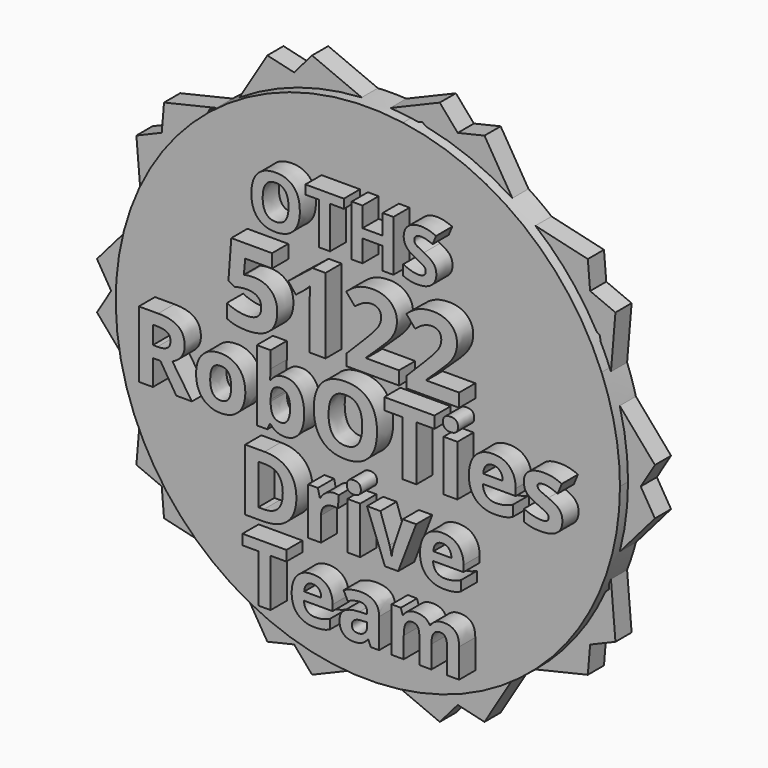
from build123d import *

# Parameters (mm, degrees)
F1_DEPTH       = 7.62
F3_DEPTH       = 5.08
F4_TEXT_SIZE   = 17.9359663485
F4_TEXT_SIZE_2 = 26.5140358048
F4_TEXT_SIZE_3 = 23.3947377031
F5_DEPTH       = 5.08
F6_DEPTH       = 12.7
F7_TEXT_SIZE   = 21.7276495985
F7_TEXT_SIZE_2 = 20.4692439487
F8_DEPTH       = 12.7


# Not quite as in the source:
# - Text() gives the source's letters only with a copy of the font that has no kerning and outlines rounded to 1/6400 em; it was checked with that copy


with BuildPart() as f1:
    # F0 (on Front) → F1 (new body)
    with BuildSketch(Plane.XZ):
        with BuildLine():
            ThreePointArc((-8.8088285315, -62.7875043569), (23.7650828926, -58.7799880791), (49.9711595476, -39.0224214643))
            Line((49.9711595476, -39.0224214643), (-8.8088285315, -62.7875043569))
        make_face()
        Polygon((-8.8088285315, -62.7875043569), (49.9711595476, -39.0224214643), (58.7799880791, 23.7650828926), (8.8088285315, 62.7875043569), (-49.9711595476, 39.0224214643), (-58.7799880791, -23.7650828926), align=None)
        with BuildLine():
            Line((58.7799880791, 23.7650828926), (49.9711595476, -39.0224214643))
            ThreePointArc((49.9711595476, -39.0224214643), (59.9506394201, -20.6346067707), (63.4024144924, 0))
            ThreePointArc((63.4024144924, 0), (62.2360800963, 12.1052260495), (58.7799880791, 23.7650828926))
        make_face()
        with BuildLine():
            ThreePointArc((-58.7799880791, -23.7650828926), (-39.0224214643, -49.9711595476), (-8.8088285315, -62.7875043569))
            Line((-8.8088285315, -62.7875043569), (-58.7799880791, -23.7650828926))
        make_face()
        with BuildLine():
            Line((8.8088285315, 62.7875043569), (58.7799880791, 23.7650828926))
            ThreePointArc((58.7799880791, 23.7650828926), (39.0224214643, 49.9711595476), (8.8088285315, 62.7875043569))
        make_face()
        with BuildLine():
            ThreePointArc((-49.9711595476, 39.0224214643), (-62.7875043569, 8.8088285315), (-58.7799880791, -23.7650828926))
            Line((-58.7799880791, -23.7650828926), (-49.9711595476, 39.0224214643))
        make_face()
        with BuildLine():
            Line((-49.9711595476, 39.0224214643), (8.8088285315, 62.7875043569))
            ThreePointArc((8.8088285315, 62.7875043569), (-23.7650828926, 58.7799880791), (-49.9711595476, 39.0224214643))
        make_face()
    extrude(amount=F1_DEPTH)

    # F2 (on Front) → F3 (join)
    with BuildSketch(Plane.XZ):
        Polygon((58.7700592924, -19.0955498129), (70.1562219705, -5.9126556007), (66.5778460996, 0), (58.3118093375, -13.6582154365), align=None)
        Polygon((60.2329475992, -36.453353768), (58.7700592924, -19.0955498129), (58.4000724019, -19.5239204743), (58.6371492593, -25.3601040719), (54.7388375906, -28.7366433033), (53.8626089435, -39.1334760668), align=None)
        Polygon((58.4000724019, -19.5239204743), (58.7700592924, -19.0955498129), (58.3118093375, -13.6582154365), (58.1712319857, -13.8904955257), align=None)
        Polygon((58.3118093375, -13.6582154365), (66.5778460996, 0), (58.3118093375, 13.6582154365), (57.4618354371, 3.5729066254), (58.022210925, -10.2220047241), align=None)
        Polygon((58.3118093375, 13.6582154365), (66.5778460996, 0), (70.1562219705, 5.9126556007), (58.7700592924, 19.0955498129), align=None)
        Polygon((56.9615185047, 15.8893406574), (58.3118093375, 13.6582154365), (58.7700592924, 19.0955498129), (56.7355910586, 21.4510562519), align=None)
        Polygon((39.1471471206, -45.324549964), (53.8626089435, -39.1334760668), (54.7388375906, -28.7366433033), (43.0687894167, -38.8447051621), align=None)
        Polygon((53.2822040713, -46.0202314936), (53.8626089435, -39.1334760668), (39.1471471206, -45.324549964), (36.3218941635, -49.992798444), align=None)
        Polygon((56.7355910586, 21.4510562519), (58.7700592924, 19.0955498129), (60.2329475992, 36.453353768), (53.8626089435, 39.1334760668), (54.5138868121, 31.4057818125), (56.3869923353, 30.0326030701), align=None)
        Polygon((36.3218941635, -49.992798444), (39.1471471206, -45.324549964), (34.3856584193, -47.3277985719), (31.0090748499, -51.2372055647), align=None)
        Polygon((27.3027344876, -64.8954210012), (36.3218941635, -49.992798444), (31.0090748499, -51.2372055647), (20.5736858937, -63.3192943739), align=None)
        Polygon((54.5138868121, 31.4057818125), (53.8626089435, 39.1334760668), (39.1471471206, 45.324549964), (42.0336708321, 40.5550620161), align=None)
        Polygon((39.1471471206, 45.324549964), (53.8626089435, 39.1334760668), (53.2822040713, 46.0202314936), (36.3218941635, 49.992798444), align=None)
        Polygon((20.5736858937, -63.3192943739), (31.0090748499, -51.2372055647), (27.9281377044, -51.9588450363), (16.7323368111, -61.656135596), (5.3557181263, -59.5412450645), (5.0296052662, -59.6784469301), align=None)
        Polygon((34.3856584193, 47.3277985719), (39.1471471206, 45.324549964), (36.3218941635, 49.992798444), (31.0090748499, 51.2372055647), align=None)
        Polygon((16.0561952124, -68.5496431262), (20.5736858937, -63.3192943739), (5.0296052662, -59.6784469301), (0, -61.7944972622), align=None)
        Polygon((31.0090748499, 51.2372055647), (36.3218941635, 49.992798444), (27.3027344876, 64.8954210012), (20.5736858937, 63.3192943739), align=None)
        Polygon((0, -61.7944972622), (5.0296052662, -59.6784469301), (0.9363181688, -58.7196875012), (-0.1077097283, -58.525604815), (-5.0296052662, -59.6784469301), align=None)
        Polygon((25.7973886351, 52.4579245566), (31.0090748499, 51.2372055647), (20.5736858937, 63.3192943739), (13.3043369244, 61.6166146692), align=None)
        Polygon((-16.0561952124, -68.5496431262), (0, -61.7944972622), (-5.0296052662, -59.6784469301), (-20.5736858937, -63.3192943739), align=None)
        Polygon((13.3043369244, 61.6166146692), (20.5736858937, 63.3192943739), (16.0561952124, 68.5496431262), (0, 61.7944972622), (3.1109304757, 60.485669806), (11.6762800979, 62.8101475469), align=None)
        Polygon((-5.0296052662, -59.6784469301), (-13.8355160958, -55.9736332222), (-29.4205419552, -53.0764082614), (-20.5736858937, -63.3192943739), align=None)
        Polygon((-29.4205419552, -53.0764082614), (-31.0090748499, -51.2372055647), (-36.3218941635, -49.992798444), (-35.0939728795, -52.0217288636), align=None)
        Polygon((-5.0296052662, 59.6784469301), (-2.2567733337, 59.0289740989), (3.1109304757, 60.485669806), (0, 61.7944972622), align=None)
        Polygon((-20.5736858937, -63.3192943739), (-29.4205419552, -53.0764082614), (-35.0939728795, -52.0217288636), (-27.3027344876, -64.8954210012), align=None)
        Polygon((-36.3218941635, -49.992798444), (-39.1471471206, -45.324549964), (-41.6306026947, -44.2797131003), (-38.9106826662, -49.3864336014), align=None)
        Polygon((-35.0939728795, -52.0217288636), (-36.3218941635, -49.992798444), (-38.9106826662, -49.3864336014), (-37.7722665333, -51.5238394603), align=None)
        Polygon((-5.0296052662, 59.6784469301), (0, 61.7944972622), (-16.0561952124, 68.5496431262), (-20.5736858937, 63.3192943739), align=None)
        Polygon((-31.0090748499, 51.2372055647), (-30.7109872532, 51.3070258063), (-14.4175277472, 55.7287698815), (-5.0296052662, 59.6784469301), (-20.5736858937, 63.3192943739), align=None)
        Polygon((-38.9106826662, -49.3864336014), (-41.6306026947, -44.2797131003), (-53.8626089435, -39.1334760668), (-53.2822040713, -46.0202314936), align=None)
        Polygon((-53.8626089435, -39.1334760668), (-41.6306026947, -44.2797131003), (-49.0502385623, -30.3491540402), (-55.203342333, -23.2250931621), align=None)
        Polygon((-31.0215692126, 51.2227395969), (-31.0090748499, 51.2372055647), (-36.3218941635, 49.992798444), (-36.4728550969, 49.7433612579), align=None)
        Polygon((-36.3218941635, 49.992798444), (-31.0090748499, 51.2372055647), (-20.5736858937, 63.3192943739), (-27.3027344876, 64.8954210012), align=None)
        Polygon((-60.2329475992, -36.453353768), (-53.8626089435, -39.1334760668), (-55.203342333, -23.2250931621), (-58.7700592924, -19.0955498129), align=None)
        Polygon((-58.7700592924, -19.0955498129), (-55.203342333, -23.2250931621), (-55.637164048, -18.0776104417), (-58.3118093375, -13.6582154365), align=None)
        Polygon((-36.4728550969, 49.7433612579), (-36.3218941635, 49.992798444), (-53.2822040713, 46.0202314936), (-53.8626089435, 39.1334760668), (-43.9909741776, 43.2866600482), (-41.826909206, 48.2903698274), align=None)
        Polygon((-50.1240356268, 29.1059122644), (-43.9909741776, 43.2866600482), (-53.8626089435, 39.1334760668), (-55.203342333, 23.2250931621), align=None)
        Polygon((-70.1562219705, -5.9126556007), (-58.7700592924, -19.0955498129), (-58.3118093375, -13.6582154365), (-66.5778460996, 0), align=None)
        Polygon((-66.5778460996, 0), (-58.3118093375, -13.6582154365), (-58.2610268923, -13.0556597083), (-63.8335827643, -2.5930413162), (-58.0660756499, 10.7424787021), (-58.3118093375, 13.6582154365), align=None)
        Polygon((-55.203342333, 23.2250931621), (-53.8626089435, 39.1334760668), (-60.2329475992, 36.453353768), (-58.7700592924, 19.0955498129), align=None)
        Polygon((-58.3118093375, 13.6582154365), (-55.637164048, 18.0776104417), (-55.203342333, 23.2250931621), (-58.7700592924, 19.0955498129), align=None)
        Polygon((-70.1562219705, 5.9126556007), (-66.5778460996, 0), (-58.3118093375, 13.6582154365), (-58.7700592924, 19.0955498129), align=None)
    extrude(amount=F3_DEPTH)

    # F4 (on Front) → F5 (join)
    with BuildSketch(Plane.XZ):
        with Locations((-26.2698885053, 31.7180491984)):
            Text('OTHS', F4_TEXT_SIZE, font='Open Sans', font_style=FontStyle.BOLD, text_align=(TextAlign.LEFT, TextAlign.BOTTOM))
        with Locations((-32.6615534723, 7.6555427804)):
            Text('5122', F4_TEXT_SIZE_2, font='Open Sans', font_style=FontStyle.BOLD, text_align=(TextAlign.LEFT, TextAlign.BOTTOM))
        with Locations((-55.6239578873, -12.7949038579)):
            Text('RobOTies', F4_TEXT_SIZE_3, font='Open Sans', font_style=FontStyle.BOLD, text_align=(TextAlign.LEFT, TextAlign.BOTTOM))
    extrude(amount=F5_DEPTH)

    # F4 (on Front) → F6 (join)
    with BuildSketch(Plane.XZ):
        with Locations((-26.2698885053, 31.7180491984)):
            Text('OTHS', F4_TEXT_SIZE, font='Open Sans', font_style=FontStyle.BOLD, text_align=(TextAlign.LEFT, TextAlign.BOTTOM))
        with Locations((-32.6615534723, 7.6555427804)):
            Text('5122', F4_TEXT_SIZE_2, font='Open Sans', font_style=FontStyle.BOLD, text_align=(TextAlign.LEFT, TextAlign.BOTTOM))
        with Locations((-55.6239578873, -12.7949038579)):
            Text('RobOTies', F4_TEXT_SIZE_3, font='Open Sans', font_style=FontStyle.BOLD, text_align=(TextAlign.LEFT, TextAlign.BOTTOM))
    extrude(amount=F6_DEPTH)

    # F7 (on Front) → F8 (join)
    with BuildSketch(Plane.XZ):
        with Locations((-28.7323780358, -33.5082784295)):
            Text('Drive', F7_TEXT_SIZE, font='Open Sans', font_style=FontStyle.BOLD, text_align=(TextAlign.LEFT, TextAlign.BOTTOM))
        with Locations((-27.86533162, -52.5523647666)):
            Text('Team', F7_TEXT_SIZE_2, font='Open Sans', font_style=FontStyle.BOLD, text_align=(TextAlign.LEFT, TextAlign.BOTTOM))
    extrude(amount=F8_DEPTH)


solid = f1.part
